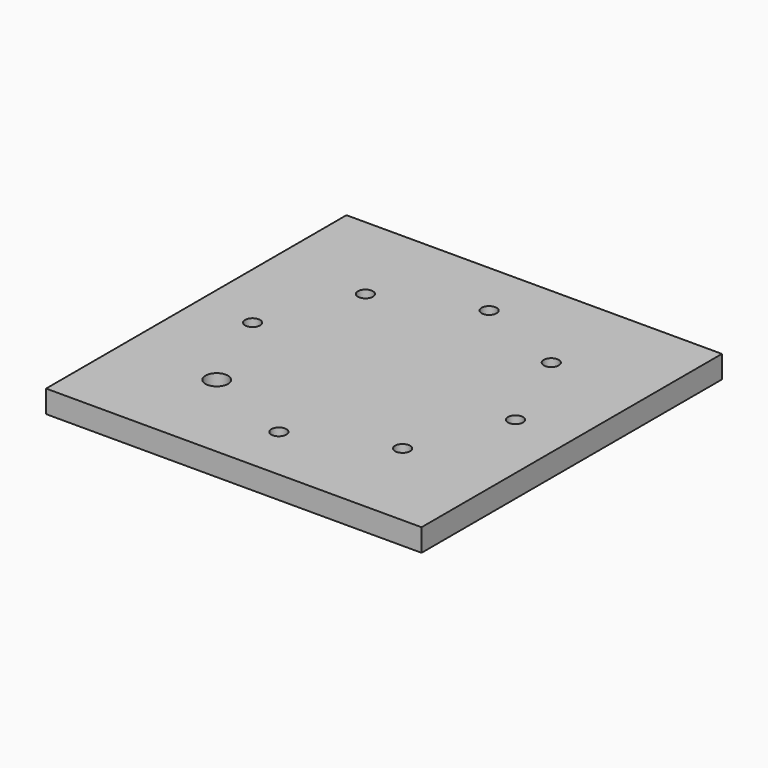
from build123d import *

# Parameters (mm, degrees)
F0_W            = 250
F0_H            = 250
F1_DEPTH        = 15
F5_R            = 5
F6_DEPTH        = 15.001
F6_COPIES_COUNT = 7
F6_COPIES_ANGLE = 270
F8_R            = 7.5
F9_DEPTH        = 15.001


# Not quite as in the source:
# - a pattern or mirror of a feature is missing from the dataset's text; its kind, count and spacing are read off the source's solid


with BuildPart() as f1:
    # F0 (on Top) → F1 (new body)
    with BuildSketch(Plane.XY):
        with Locations((-125, 125)):
            Rectangle(F0_W, F0_H)
    extrude(amount=F1_DEPTH)

    # F5 (on face) → F6 (cut, through all)
    with BuildSketch(Plane.XY.offset(15)):
        with Locations((-212.5, 125)):
            Circle(F5_R)
    f6 = extrude(amount=-F6_DEPTH, mode=Mode.SUBTRACT)

    # F6_copies: F6 ×7 about axis
    f6_copies_axis = Axis((-125, 125, 0), (0, 0, -1))
    for i in range(1, F6_COPIES_COUNT):
        add(f6.rotate(f6_copies_axis, i * F6_COPIES_ANGLE / (F6_COPIES_COUNT - 1)), mode=Mode.SUBTRACT)

    # F8 (on face) → F9 (cut, through all)
    with BuildSketch(Plane.XY.offset(15)):
        with Locations((-186.8718433538, 63.1281566462)):
            Circle(F8_R)
    extrude(amount=-F9_DEPTH, mode=Mode.SUBTRACT)


solid = f1.part
